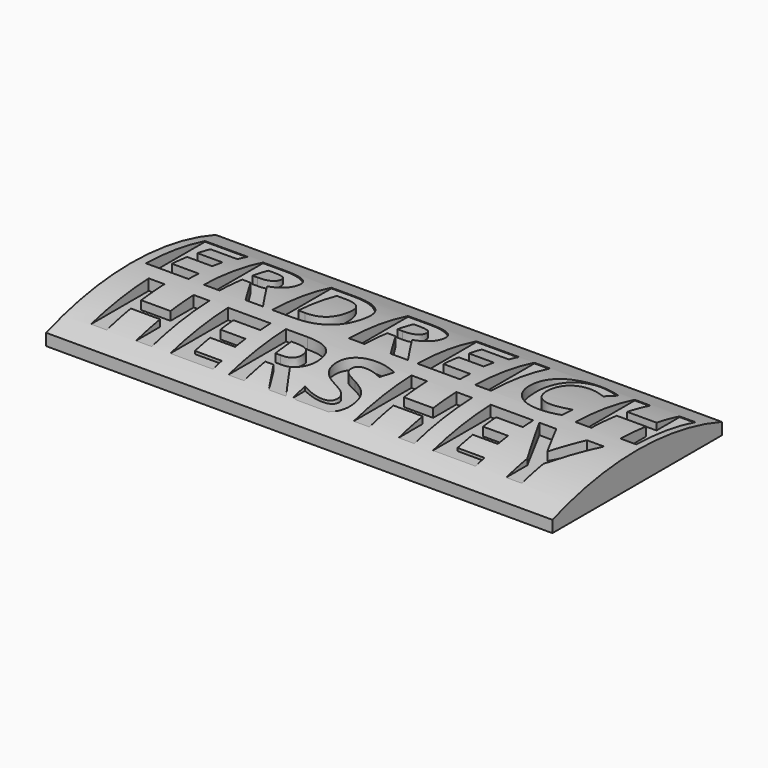
from build123d import *

# Parameters (mm, degrees)
F0_W         = 136.525
F0_H         = 57.15
F1_DEPTH     = 3.175
F3_DEPTH     = 136.525
F5_TEXT_SIZE = 27.9272541311
F6_DEPTH     = 3.81


# Not quite as in the source:
# - Text() gives the source's letters only with a copy of the font that has no kerning and outlines rounded to 1/6400 em; it was checked with that copy


with BuildPart() as f1:
    # F0 (on Top) → F1 (new body)
    with BuildSketch(Plane.XY):
        with Locations((68.2625, 28.575)):
            Rectangle(F0_W, F0_H)
    extrude(amount=F1_DEPTH)

    # F2 (on Right) → F3 (join)
    with BuildSketch(Plane.YZ):
        with BuildLine():
            Line((55.1439449191, 1.8612246495), (57.1475178003, 3.183264751))
            ThreePointArc((57.1475178003, 3.183264751), (28.5718578405, 8.1030729003), (0, 3.1612317543))
            Line((0, 3.1612317543), (1.2994168792, 1.8612246495))
            Line((1.2994168792, 1.8612246495), (55.1439449191, 1.8612246495))
        make_face()
    extrude(amount=F3_DEPTH)

    # F5 (on offset) → F6 (cut)
    with BuildSketch(Plane.XY.offset(8.89)):
        with Locations((2.5511e-06, 30.5050779134)):
            Text('ERDREICH', F5_TEXT_SIZE, font='Open Sans', font_style=FontStyle.BOLD, text_align=(TextAlign.LEFT, TextAlign.BOTTOM))
        with Locations((4.7258175861, 5.6254728697)):
            Text('HERSHEY', F5_TEXT_SIZE, font='Open Sans', font_style=FontStyle.BOLD, text_align=(TextAlign.LEFT, TextAlign.BOTTOM))
    extrude(amount=-F6_DEPTH, mode=Mode.SUBTRACT)


solid = f1.part
